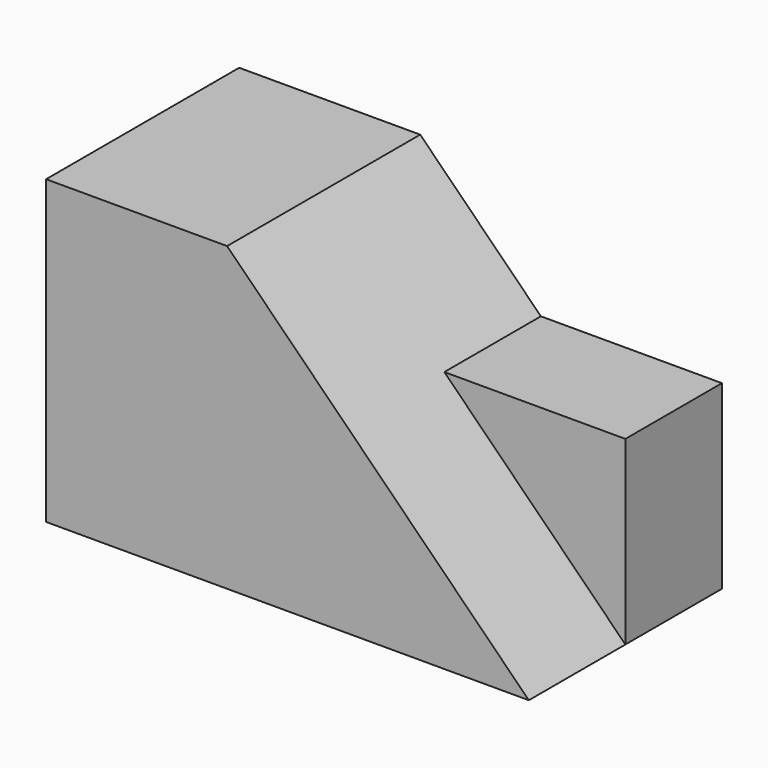
from build123d import *

# Parameters (mm, degrees)
F0_W      = 50.8
F0_H      = 31.75
F1_DEPTH  = 25.4
F3_DEPTH  = 25.4
F4_DEPTH  = 25.4
F6_DEPTH  = 25.4
F8_DEPTH  = 12.7
F10_DEPTH = 25.4


# Not quite as in the source:
# - a feature names something its author has since deleted; it is built from what else it names


with BuildPart() as f1:
    # F0 (on Front) → F1 (new body)
    with BuildSketch(Plane.XZ):
        with Locations((25.4, 15.875)):
            Rectangle(F0_W, F0_H)
    extrude(amount=F1_DEPTH)

    # F2 (on face) → F3 (cut)
    with BuildSketch(Plane.XZ.offset(25.4)):
        Polygon((25.4, 31.75), (50.8, 0), (50.8, 31.75), align=None)
    extrude(amount=-F3_DEPTH, mode=Mode.SUBTRACT)

    # F4 (add): a face of the model
    f4_faces = [f1.faces().sort_by_distance(p)[0] for p in [
        (38.1, -12.7, 15.875),
    ]]
    extrude(f4_faces, amount=F4_DEPTH)

    # F5 (on face) → F6 (cut)
    with BuildSketch(Plane.XZ.offset(25.4)):
        Polygon((45.2340677599, 47.6172542079), (25.4, 31.75), (50.8, 31.75), (50.8, 0), (70.6340677599, 15.8672542079), align=None)
    extrude(amount=-F6_DEPTH, mode=Mode.SUBTRACT)

    # F7 (on face) → F8 (cut)
    with BuildSketch(Plane.XZ.offset(25.4)):
        Polygon((19.05, 31.75), (50.8, 0), (50.8, 31.75), align=None)
    extrude(amount=-F8_DEPTH, mode=Mode.SUBTRACT)

    # F9 (on face) → F10 (cut)
    with BuildSketch(Plane.XZ.offset(12.7)):
        Polygon((31.75, 19.05), (50.8, 19.05), (50.8, 31.75), (19.05, 31.75), align=None)
    extrude(amount=-F10_DEPTH, mode=Mode.SUBTRACT)


solid = f1.part
